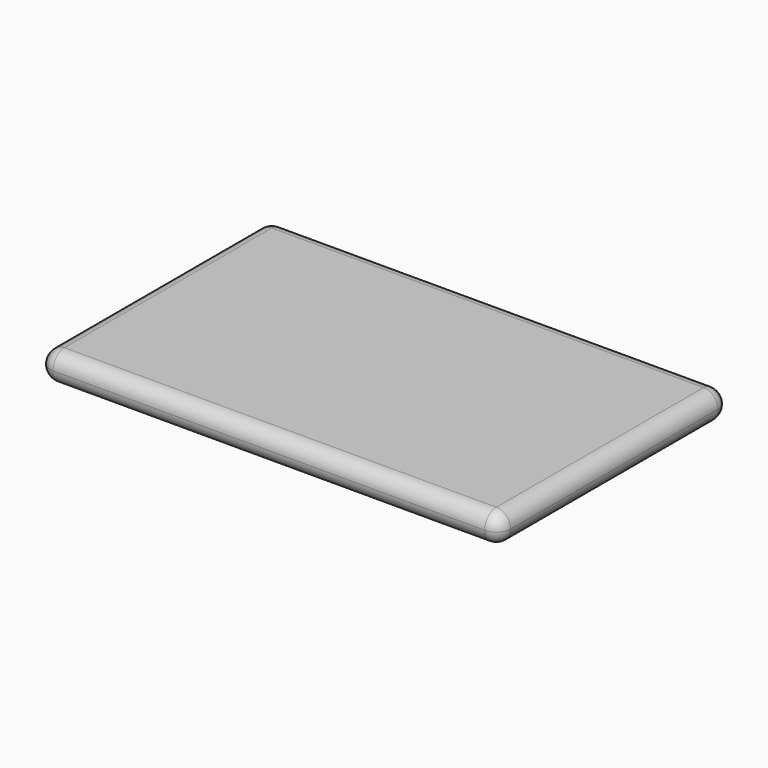
from build123d import *

# Parameters (mm, degrees)
F0_W     = 20.32
F0_H     = 12.7
F1_DEPTH = 1.27
F2_R     = 0.63499
F3_R     = 0.635
F4_R     = 0.63499
F5_R     = 0.63499
F6_R     = 0.63499
F7_W     = 17.7417555824
F7_H     = 10.0744650699
F8_DEPTH = 1.27


# Not quite as in the source:
# - a fillet or chamfer is up to 0.001 mm smaller than in the source, because OpenCascade refuses the exact size


with BuildPart() as f1:
    # F0 (on Top) → F1 (new body)
    with BuildSketch(Plane.XY):
        with Locations((-10.16, 6.35)):
            Rectangle(F0_W, F0_H)
    extrude(amount=F1_DEPTH)

    # F2 (radius 0.635 in the source; OpenCascade refuses exactly that, so slightly less here)
    f2_edges = [f1.edges().sort_by_distance(p)[0] for p in [
        (0, 6.35, 1.27),
        (0, 6.35, 0),
    ]]
    fillet(f2_edges, radius=F2_R)

    # F3
    f3_edges = [f1.edges().sort_by_distance(p)[0] for p in [
        (-20.32, 6.35, 1.27),
    ]]
    fillet(f3_edges, radius=F3_R)

    # F4 (radius 0.635 in the source; OpenCascade refuses exactly that, so slightly less here)
    f4_edges = [f1.edges().sort_by_distance(p)[0] for p in [
        (-20.32, 6.35, 0),
    ]]
    fillet(f4_edges, radius=F4_R)

    # F5 (radius 0.635 in the source; OpenCascade refuses exactly that, so slightly less here)
    f5_edges = [f1.edges().sort_by_distance(p)[0] for p in [
        (-10.159995, 12.7, 1.27),
    ]]
    fillet(f5_edges, radius=F5_R)

    # F6 (radius 0.635 in the source; OpenCascade refuses exactly that, so slightly less here)
    f6_edges = [f1.edges().sort_by_distance(p)[0] for p in [
        (-10.159995, 0, 1.27),
    ]]
    fillet(f6_edges, radius=F6_R)

    # F7 (on Top) → F8 (join)
    with BuildSketch(Plane.XY):
        with Locations((-10.1206521504, 6.3767505344)):
            Rectangle(F7_W, F7_H)
    extrude(amount=F8_DEPTH)


solid = f1.part
